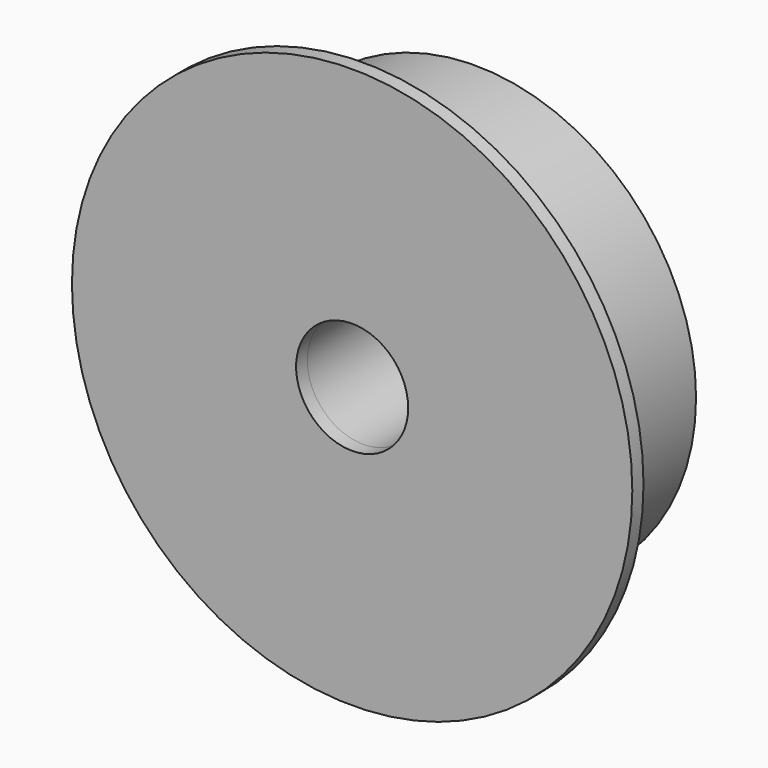
from build123d import *

# Parameters (mm, degrees)
F0_R     = 20
F0_R_2   = 15.75
F0_R_3   = 4
F1_DEPTH = 1
F2_DEPTH = 10


# Not quite as in the source:
# - a feature names something its author has since deleted; it is built from what else it names


with BuildPart() as f1:
    # F0 (on Front) → F1 (new body)
    with BuildSketch(Plane.XZ):
        Circle(F0_R)
        Circle(F0_R_2, mode=Mode.SUBTRACT)
        Circle(F0_R_2)
        Circle(F0_R_3, mode=Mode.SUBTRACT)
    extrude(amount=F1_DEPTH)

    # F0 (on Front) → F2 (join)
    with BuildSketch(Plane.XZ):
        Circle(F0_R_2)
        Circle(F0_R_3, mode=Mode.SUBTRACT)
    extrude(amount=-F2_DEPTH)


solid = f1.part
